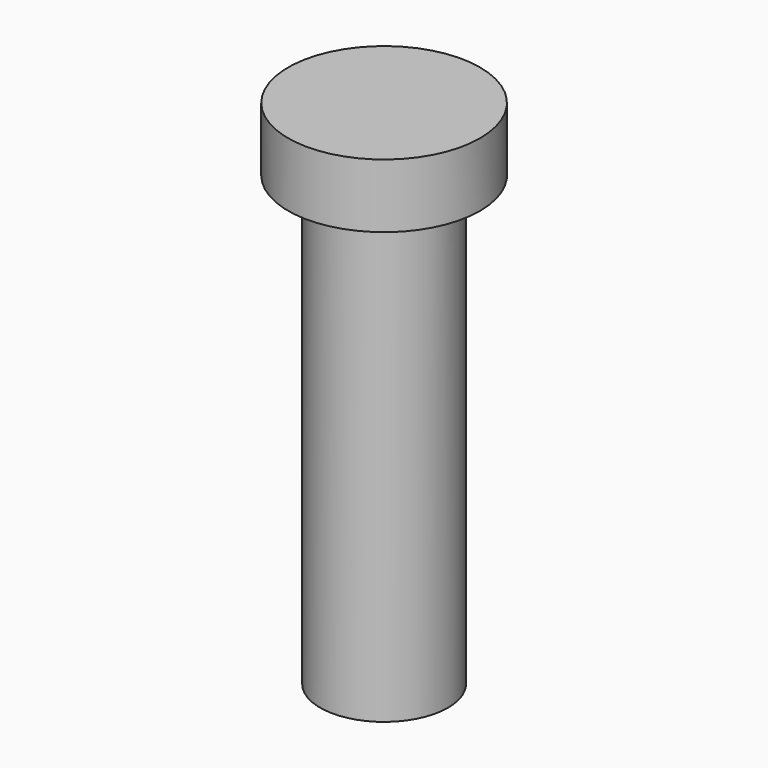
from build123d import *

# Parameters (mm, degrees)
F2_R     = 12.7
F3_DEPTH = 44.45
F4_R     = 19.05
F5_DEPTH = 12.7


# Not quite as in the source:
# - a variable given as a bare number and used for a length is read in inches; the dataset says mm whatever the document's units were


with BuildPart() as f3:
    # F2 (on Top) → F3 (new body, symmetric)
    with BuildSketch(Plane.XY):
        Circle(F2_R)
    extrude(amount=F3_DEPTH, both=True)

    # F4 (on face) → F5 (join)
    with BuildSketch(Plane.XY.offset(44.45)):
        Circle(F4_R)
    extrude(amount=F5_DEPTH)


solid = f3.part
